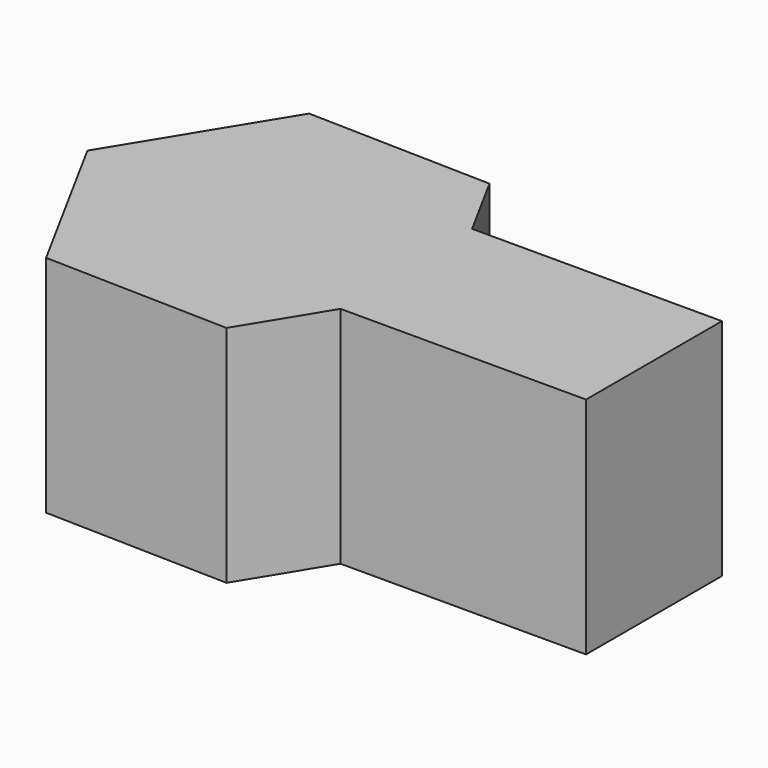
from build123d import *

# Parameters (mm, degrees)
F1_DEPTH = 25.4


# Not quite as in the source:
# - a feature of the source that left no trace in its solid (it failed there, or was rolled back) is left out


with BuildPart() as f1:
    # F0 (on Top) → F1 (new body)
    with BuildSketch(Plane.XY):
        Polygon((-36.8466593381, 18.4331755623), (-31.2554423525, 27.5824405253), (-3.4660941456, 27.5824405253), (-3.4660941456, 46.8057003116), (-31.7457578, 46.8057003116), (-35.9461061545, 54.5191512435), (-56.780353928, 55.0390858665), (-67.6477544065, 37.2560653374), (-57.6809071116, 18.9531101853), align=None)
    extrude(amount=F1_DEPTH)


solid = f1.part
